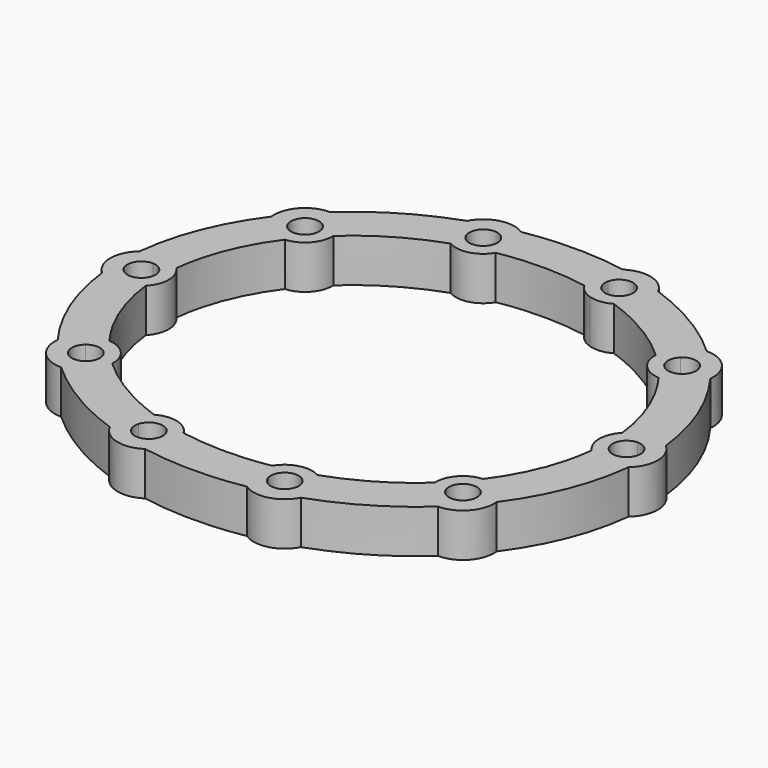
from build123d import *

# Parameters (mm, degrees)
F1_DEPTH = 3.5


with BuildPart() as f1:
    # F0 (on Top) → F1 (new body)
    with BuildSketch(Plane.XY):
        with BuildLine():
            add(Edge.make_bspline(
                [(17.9176777417, -1.5284816882), (18, -0.7659924616), (18, 0)],
                knots=[6.1875093004, 6.1875093004, 6.1875093004, 6.2831853072, 6.2831853072, 6.2831853072], degree=2, weights=[1, 0.9988559809, 1]))
            add(Edge.make_bspline(
                [(18, 0), (18, 0.7659924616), (17.9176777417, 1.5284816882)],
                knots=[0, 0, 0, 0.0956760068, 0.0956760068, 0.0956760068], degree=2, weights=[1, 0.9988559809, 1]))
            ThreePointArc((17.9176777417, 1.5284816882), (17.3, 0), (17.9176777417, -1.5284816882))
        make_face()
        with BuildLine():
            add(Edge.make_bspline(
                [(18, 0), (18, 0.7659924616), (17.9176777417, 1.5284816882)],
                knots=[0, 0, 0, 0.0956760068, 0.0956760068, 0.0956760068], degree=2, weights=[1, 0.9988559809, 1]))
            add(Edge.make_bspline(
                [(17.9176777417, -1.5284816882), (18, -0.7659924616), (18, 0)],
                knots=[6.1875093004, 6.1875093004, 6.1875093004, 6.2831853072, 6.2831853072, 6.2831853072], degree=2, weights=[1, 0.9988559809, 1]))
            add(Edge.make_bspline(
                [(15.0214595009, -8.8155084204), (17.4897174963, -5.4923559002), (17.9176777417, -1.5284816882)],
                knots=[5.6996600441, 5.6996600441, 5.6996600441, 6.1875093004, 6.1875093004, 6.1875093004], degree=2, weights=[1, 0.9703976022, 1]))
            add(Edge.make_bspline(
                [(12.9579027327, -11.1055188334), (14.108288617, -10.0449609858), (15.0214595009, -8.8155084204)],
                knots=[5.5160234188, 5.5160234188, 5.5160234188, 5.6996600441, 5.6996600441, 5.6996600441], degree=2, weights=[1, 0.9957876594, 1]))
            add(Edge.make_bspline(
                [(6.5641116037, -14.8981712717), (10.2272761366, -13.6229240841), (12.9579027327, -11.1055188334)],
                knots=[5.0856704323, 5.0856704323, 5.0856704323, 5.5160234188, 5.5160234188, 5.5160234188], degree=2, weights=[1, 0.9769387246, 1]))
            add(Edge.make_bspline(
                [(3.5634097577, -15.6833382916), (5.1022815412, -15.4070740686), (6.5641116037, -14.8981712717)],
                knots=[4.9116726299, 4.9116726299, 4.9116726299, 5.0856704323, 5.0856704323, 5.0856704323], degree=2, weights=[1, 0.9962179819, 1]))
            add(Edge.make_bspline(
                [(-3.5634097577, -15.6833382916), (0, -16.3230554133), (3.5634097577, -15.6833382916)],
                knots=[4.5131053308, 4.5131053308, 4.5131053308, 4.9116726299, 4.9116726299, 4.9116726299], degree=2, weights=[1, 0.9802086432, 1]))
            add(Edge.make_bspline(
                [(-6.5641116037, -14.8981712717), (-5.1022815412, -15.4070740686), (-3.5634097577, -15.6833382916)],
                knots=[4.3391075285, 4.3391075285, 4.3391075285, 4.5131053308, 4.5131053308, 4.5131053308], degree=2, weights=[1, 0.9962179819, 1]))
            add(Edge.make_bspline(
                [(-12.9579027327, -11.1055188334), (-10.2272761366, -13.6229240841), (-6.5641116037, -14.8981712717)],
                knots=[3.9087545419, 3.9087545419, 3.9087545419, 4.3391075285, 4.3391075285, 4.3391075285], degree=2, weights=[1, 0.9769387246, 1]))
            add(Edge.make_bspline(
                [(-15.0214595009, -8.8155084204), (-14.108288617, -10.0449609858), (-12.9579027327, -11.1055188334)],
                knots=[3.7251179166, 3.7251179166, 3.7251179166, 3.9087545419, 3.9087545419, 3.9087545419], degree=2, weights=[1, 0.9957876594, 1]))
            add(Edge.make_bspline(
                [(-17.9176777417, -1.5284816882), (-17.4897174963, -5.4923559002), (-15.0214595009, -8.8155084204)],
                knots=[3.2372686604, 3.2372686604, 3.2372686604, 3.7251179166, 3.7251179166, 3.7251179166], degree=2, weights=[1, 0.9703976022, 1]))
            add(Edge.make_bspline(
                [(-17.9176777417, 1.5284816882), (-18.0827004855, 0), (-17.9176777417, -1.5284816882)],
                knots=[3.0459166468, 3.0459166468, 3.0459166468, 3.2372686604, 3.2372686604, 3.2372686604], degree=2, weights=[1, 0.9954265412, 1]))
            add(Edge.make_bspline(
                [(-15.0214595009, 8.8155084204), (-17.4897174963, 5.4923559002), (-17.9176777417, 1.5284816882)],
                knots=[2.5580673905, 2.5580673905, 2.5580673905, 3.0459166468, 3.0459166468, 3.0459166468], degree=2, weights=[1, 0.9703976022, 1]))
            add(Edge.make_bspline(
                [(-12.9579027327, 11.1055188334), (-14.108288617, 10.0449609858), (-15.0214595009, 8.8155084204)],
                knots=[2.3744307652, 2.3744307652, 2.3744307652, 2.5580673905, 2.5580673905, 2.5580673905], degree=2, weights=[1, 0.9957876594, 1]))
            add(Edge.make_bspline(
                [(-6.5641116037, 14.8981712717), (-10.2272761366, 13.6229240841), (-12.9579027327, 11.1055188334)],
                knots=[1.9440777787, 1.9440777787, 1.9440777787, 2.3744307652, 2.3744307652, 2.3744307652], degree=2, weights=[1, 0.9769387246, 1]))
            add(Edge.make_bspline(
                [(-3.5634097577, 15.6833382916), (-5.1022815412, 15.4070740686), (-6.5641116037, 14.8981712717)],
                knots=[1.7700799764, 1.7700799764, 1.7700799764, 1.9440777787, 1.9440777787, 1.9440777787], degree=2, weights=[1, 0.9962179819, 1]))
            add(Edge.make_bspline(
                [(3.5634097577, 15.6833382916), (0, 16.3230554133), (-3.5634097577, 15.6833382916)],
                knots=[1.3715126772, 1.3715126772, 1.3715126772, 1.7700799764, 1.7700799764, 1.7700799764], degree=2, weights=[1, 0.9802086432, 1]))
            add(Edge.make_bspline(
                [(4.9945744172, 15.3717194589), (4.2861725259, 15.55358512), (3.5634097577, 15.6833382916)],
                knots=[1.2896300089, 1.2896300089, 1.2896300089, 1.3715126772, 1.3715126772, 1.3715126772], degree=2, weights=[1, 0.9991620206, 1]))
            Line((4.9945744172, 15.3717194589), (5.1111125116, 15.7303868336))
            ThreePointArc((5.1111125116, 15.7303868336), (4.4788764697, 16.247641173), (4.3632618671, 17.0562867863))
            add(Edge.make_bspline(
                [(4.3632618671, 17.0562867863), (0, 17.9552562546), (-4.3632618671, 17.0562867863)],
                knots=[1.3451287946, 1.3451287946, 1.3451287946, 1.796463859, 1.796463859, 1.796463859], degree=2, weights=[1, 0.9746449592, 1]))
            ThreePointArc((-4.3632618671, 17.0562867863), (-4.3411572816, 16.929153578), (-4.3337566303, 16.8003254145))
            ThreePointArc((-4.3337566303, 16.8003254145), (-5.3003624846, 15.6865317645), (-6.5391544874, 16.4866927147))
            add(Edge.make_bspline(
                [(-6.5391544874, 16.4866927147), (-11.1035556063, 15.028621514), (-14.3767828617, 11.8229512564)],
                knots=[1.9127637636, 1.9127637636, 1.9127637636, 2.3998182175, 2.3998182175, 2.3998182175], degree=2, weights=[1, 0.9704935031, 1]))
            ThreePointArc((-14.3767828617, 11.8229512564), (-14.1209684499, 11.4524934232), (-14.0308884413, 11.0113975023))
            ThreePointArc((-14.0308884413, 11.0113975023), (-14.6826870776, 9.9907577669), (-15.8828092758, 10.1527875208))
            add(Edge.make_bspline(
                [(-15.8828092758, 10.1527875208), (-19.1031132717, 6.0954067268), (-19.4597166867, 1.1242785485)],
                knots=[2.5226684132, 2.5226684132, 2.5226684132, 3.0773038895, 3.0773038895, 3.0773038895], degree=2, weights=[1, 0.9617932385, 1]))
            ThreePointArc((-19.4597166867, 1.1242785485), (-18.6903878313, 0.7811229969), (-18.375, 0))
            ThreePointArc((-18.375, 0), (-18.6903878313, -0.7811229969), (-19.4597166867, -1.1242785485))
            add(Edge.make_bspline(
                [(-19.4597166867, -1.1242785485), (-19.1031132717, -6.0954067268), (-15.8828092758, -10.1527875208)],
                knots=[3.2058814177, 3.2058814177, 3.2058814177, 3.7605168939, 3.7605168939, 3.7605168939], degree=2, weights=[1, 0.9617932385, 1]))
            ThreePointArc((-15.8828092758, -10.1527875208), (-14.6826870776, -9.9907577669), (-14.0308884413, -11.0113975023))
            ThreePointArc((-14.0308884413, -11.0113975023), (-14.1209684499, -11.4524934232), (-14.3767828617, -11.8229512564))
            add(Edge.make_bspline(
                [(-14.3767828617, -11.8229512564), (-11.1035556063, -15.028621514), (-6.5391544874, -16.4866927147)],
                knots=[3.8833670897, 3.8833670897, 3.8833670897, 4.3704215436, 4.3704215436, 4.3704215436], degree=2, weights=[1, 0.9704935031, 1]))
            ThreePointArc((-6.5391544874, -16.4866927147), (-5.3003624846, -15.6865317645), (-4.3337566303, -16.8003254145))
            ThreePointArc((-4.3337566303, -16.8003254145), (-4.3411572816, -16.929153578), (-4.3632618671, -17.0562867863))
            add(Edge.make_bspline(
                [(-4.3632618671, -17.0562867863), (0, -17.9552562546), (4.3632618671, -17.0562867863)],
                knots=[4.4867214482, 4.4867214482, 4.4867214482, 4.9380565126, 4.9380565126, 4.9380565126], degree=2, weights=[1, 0.9746449592, 1]))
            ThreePointArc((4.3632618671, -17.0562867863), (5.1738595774, -15.7119970315), (6.5391544874, -16.4866927147))
            add(Edge.make_bspline(
                [(6.5391544874, -16.4866927147), (11.1035556063, -15.028621514), (14.3767828617, -11.8229512564)],
                knots=[5.0543564172, 5.0543564172, 5.0543564172, 5.5414108711, 5.5414108711, 5.5414108711], degree=2, weights=[1, 0.9704935031, 1]))
            ThreePointArc((14.3767828617, -11.8229512564), (14.3203990411, -10.2580168136), (15.8828092758, -10.1527875208))
            add(Edge.make_bspline(
                [(15.8828092758, -10.1527875208), (19.1031132717, -6.0954067268), (19.4597166867, -1.1242785485)],
                knots=[5.6642610668, 5.6642610668, 5.6642610668, 6.2188965431, 6.2188965431, 6.2188965431], degree=2, weights=[1, 0.9617932385, 1]))
            ThreePointArc((19.4597166867, -1.1242785485), (18.375, 0), (19.4597166867, 1.1242785485))
            add(Edge.make_bspline(
                [(19.4597166867, 1.1242785485), (19.1031132717, 6.0954067268), (15.8828092758, 10.1527875208)],
                knots=[0.0642887641, 0.0642887641, 0.0642887641, 0.6189242404, 0.6189242404, 0.6189242404], degree=2, weights=[1, 0.9617932385, 1]))
            ThreePointArc((15.8828092758, 10.1527875208), (15.0212422242, 9.8944841681), (14.2457443226, 10.3501390935))
            Line((14.2457443226, 10.3501390935), (13.9368407211, 10.1257074899))
            add(Edge.make_bspline(
                [(15.0214595009, 8.8155084204), (14.5166626583, 9.4951443835), (13.9368407211, 10.1257074899)],
                knots=[0.583525263, 0.583525263, 0.583525263, 0.6852372416, 0.6852372416, 0.6852372416], degree=2, weights=[1, 0.9987071129, 1]))
            add(Edge.make_bspline(
                [(17.9176777417, 1.5284816882), (17.4897174963, 5.4923559002), (15.0214595009, 8.8155084204)],
                knots=[0.0956760068, 0.0956760068, 0.0956760068, 0.583525263, 0.583525263, 0.583525263], degree=2, weights=[1, 0.9703976022, 1]))
        make_face()
        with BuildLine():
            ThreePointArc((13.3760510537, 9.7182699473), (14.0976595024, 9.0826280726), (15.0214595009, 8.8155084204))
            add(Edge.make_bspline(
                [(15.0214595009, 8.8155084204), (14.5166626583, 9.4951443835), (13.9368407211, 10.1257074899)],
                knots=[0.583525263, 0.583525263, 0.583525263, 0.6852372416, 0.6852372416, 0.6852372416], degree=2, weights=[1, 0.9987071129, 1]))
            Line((13.9368407211, 10.1257074899), (13.3760510537, 9.7182699473))
        make_face()
        with BuildLine():
            add(Edge.make_bspline(
                [(12.9579027327, -11.1055188334), (14.108288617, -10.0449609858), (15.0214595009, -8.8155084204)],
                knots=[5.5160234188, 5.5160234188, 5.5160234188, 5.6996600441, 5.6996600441, 5.6996600441], degree=2, weights=[1, 0.9957876594, 1]))
            ThreePointArc((15.0214595009, -8.8155084204), (13.5215456234, -9.5386709311), (12.9579027327, -11.1055188334))
        make_face()
        with BuildLine():
            Line((13.3760510537, 9.7182699473), (13.9368407211, 10.1257074899))
            add(Edge.make_bspline(
                [(13.9368407211, 10.1257074899), (13.4699604962, 10.6334451693), (12.9579027327, 11.1055188334)],
                knots=[0.6852372416, 0.6852372416, 0.6852372416, 0.7671618883, 0.7671618883, 0.7671618883], degree=2, weights=[1, 0.9991611613, 1]))
            ThreePointArc((12.9579027327, 11.1055188334), (13.0494972112, 10.376483346), (13.3760510537, 9.7182699473))
        make_face()
        with BuildLine():
            add(Edge.make_bspline(
                [(13.9368407211, 10.1257074899), (13.4699604962, 10.6334451693), (12.9579027327, 11.1055188334)],
                knots=[0.6852372416, 0.6852372416, 0.6852372416, 0.7671618883, 0.7671618883, 0.7671618883], degree=2, weights=[1, 0.9991611613, 1]))
            Line((13.9368407211, 10.1257074899), (14.2457443226, 10.3501390935))
            ThreePointArc((14.2457443226, 10.3501390935), (14.0353149039, 11.1110967871), (14.3767828617, 11.8229512564))
            add(Edge.make_bspline(
                [(14.3767828617, 11.8229512564), (11.1035556063, 15.028621514), (6.5391544874, 16.4866927147)],
                knots=[0.7417744361, 0.7417744361, 0.7417744361, 1.22882889, 1.22882889, 1.22882889], degree=2, weights=[1, 0.9704935031, 1]))
            ThreePointArc((6.5391544874, 16.4866927147), (5.9852845562, 15.8061456806), (5.1111125116, 15.7303868336))
            Line((5.1111125116, 15.7303868336), (4.9945744172, 15.3717194589))
            add(Edge.make_bspline(
                [(6.5641116037, 14.8981712717), (5.7916200863, 15.1670965756), (4.9945744172, 15.3717194589)],
                knots=[1.1975148749, 1.1975148749, 1.1975148749, 1.2896300089, 1.2896300089, 1.2896300089], degree=2, weights=[1, 0.9989395377, 1]))
            add(Edge.make_bspline(
                [(12.9579027327, 11.1055188334), (10.2272761366, 13.6229240841), (6.5641116037, 14.8981712717)],
                knots=[0.7671618883, 0.7671618883, 0.7671618883, 1.1975148749, 1.1975148749, 1.1975148749], degree=2, weights=[1, 0.9769387246, 1]))
        make_face()
        with BuildLine():
            add(Edge.make_bspline(
                [(3.5634097577, -15.6833382916), (5.1022815412, -15.4070740686), (6.5641116037, -14.8981712717)],
                knots=[4.9116726299, 4.9116726299, 4.9116726299, 5.0856704323, 5.0856704323, 5.0856704323], degree=2, weights=[1, 0.9962179819, 1]))
            ThreePointArc((6.5641116037, -14.8981712718), (4.9018512412, -14.6719794869), (3.5634097577, -15.6833382916))
        make_face()
        with BuildLine():
            ThreePointArc((4.7789192427, 14.7080010786), (5.6917962826, 14.6127028418), (6.5641116037, 14.8981712718))
            add(Edge.make_bspline(
                [(6.5641116037, 14.8981712717), (5.7916200863, 15.1670965756), (4.9945744172, 15.3717194589)],
                knots=[1.1975148749, 1.1975148749, 1.1975148749, 1.2896300089, 1.2896300089, 1.2896300089], degree=2, weights=[1, 0.9989395377, 1]))
            Line((4.9945744172, 15.3717194589), (4.7789192427, 14.7080010786))
        make_face()
        with BuildLine():
            add(Edge.make_bspline(
                [(14.3767828617, 11.8229512564), (11.1035556063, 15.028621514), (6.5391544874, 16.4866927147)],
                knots=[0.7417744361, 0.7417744361, 0.7417744361, 1.22882889, 1.22882889, 1.22882889], degree=2, weights=[1, 0.9704935031, 1]))
            ThreePointArc((14.3767828617, 11.8229512564), (15.2555877261, 12.1319710397), (16.06603256, 11.6726559111))
            Line((16.06603256, 11.6726559111), (16.5770547092, 12.0439352353))
            add(Edge.make_bspline(
                [(16.5770547092, 12.0439352353), (15.897962477, 12.8109634173), (15.1361324024, 13.5113194409)],
                knots=[0.6759759799, 0.6759759799, 0.6759759799, 0.7780428717, 0.7780428717, 0.7780428717], degree=2, weights=[1, 0.9986980763, 1]))
            add(Edge.make_bspline(
                [(15.1361324024, 13.5113194409), (11.9335945642, 16.455436168), (7.6791841945, 17.9491080015)],
                knots=[0.7780428717, 0.7780428717, 0.7780428717, 1.2010559415, 1.2010559415, 1.2010559415], degree=2, weights=[1, 0.9777157528, 1]))
            add(Edge.make_bspline(
                [(7.6791841945, 17.9491080015), (6.8516175805, 18.2396565932), (6.0001876976, 18.4666788968)],
                knots=[1.2010559415, 1.2010559415, 1.2010559415, 1.2845411506, 1.2845411506, 1.2845411506], degree=2, weights=[1, 0.999128904, 1]))
            Line((6.0001876976, 18.4666788968), (5.806400749, 17.8702639953))
            ThreePointArc((5.806400749, 17.8702639953), (6.368900749, 17.4615838233), (6.5837566303, 16.8003254145))
            ThreePointArc((6.5837566303, 16.8003254145), (6.5725502802, 16.6419312688), (6.5391544874, 16.4866927147))
        make_face()
        with BuildLine():
            ThreePointArc((16.2808884413, 11.0113975023), (16.1765281767, 10.5381961386), (15.8828092758, 10.1527875208))
            add(Edge.make_bspline(
                [(19.4597166867, 1.1242785485), (19.1031132717, 6.0954067268), (15.8828092758, 10.1527875208)],
                knots=[0.0642887641, 0.0642887641, 0.0642887641, 0.6189242404, 0.6189242404, 0.6189242404], degree=2, weights=[1, 0.9617932385, 1]))
            ThreePointArc((19.4597166867, 1.1242785485), (20.2811229969, 0.8096121687), (20.625, 0))
            ThreePointArc((20.625, 0), (20.2811229969, -0.8096121687), (19.4597166867, -1.1242785485))
            add(Edge.make_bspline(
                [(15.8828092758, -10.1527875208), (19.1031132717, -6.0954067268), (19.4597166867, -1.1242785485)],
                knots=[5.6642610668, 5.6642610668, 5.6642610668, 6.2188965431, 6.2188965431, 6.2188965431], degree=2, weights=[1, 0.9617932385, 1]))
            ThreePointArc((15.8828092758, -10.1527875208), (16.1765281767, -10.5381961386), (16.2808884413, -11.0113975023))
            ThreePointArc((16.2808884413, -11.0113975023), (15.5969843622, -12.0463174937), (14.3767828617, -11.8229512564))
            add(Edge.make_bspline(
                [(6.5391544874, -16.4866927147), (11.1035556063, -15.028621514), (14.3767828617, -11.8229512564)],
                knots=[5.0543564172, 5.0543564172, 5.0543564172, 5.5414108711, 5.5414108711, 5.5414108711], degree=2, weights=[1, 0.9704935031, 1]))
            ThreePointArc((6.5391544874, -16.4866927147), (6.5725502802, -16.6419312688), (6.5837566303, -16.8003254145))
            ThreePointArc((6.5837566303, -16.8003254145), (5.5875847938, -17.9179247632), (4.3632618671, -17.0562867863))
            add(Edge.make_bspline(
                [(-4.3632618671, -17.0562867863), (0, -17.9552562546), (4.3632618671, -17.0562867863)],
                knots=[4.4867214482, 4.4867214482, 4.4867214482, 4.9380565126, 4.9380565126, 4.9380565126], degree=2, weights=[1, 0.9746449592, 1]))
            ThreePointArc((-4.3632618671, -17.0562867863), (-5.7436536832, -17.8886537975), (-6.5391544874, -16.4866927147))
            add(Edge.make_bspline(
                [(-14.3767828617, -11.8229512564), (-11.1035556063, -15.028621514), (-6.5391544874, -16.4866927147)],
                knots=[3.8833670897, 3.8833670897, 3.8833670897, 4.3704215436, 4.3704215436, 4.3704215436], degree=2, weights=[1, 0.9704935031, 1]))
            ThreePointArc((-14.3767828617, -11.8229512564), (-15.9913778415, -11.764778191), (-15.8828092758, -10.1527875208))
            add(Edge.make_bspline(
                [(-19.4597166867, -1.1242785485), (-19.1031132717, -6.0954067268), (-15.8828092758, -10.1527875208)],
                knots=[3.2058814177, 3.2058814177, 3.2058814177, 3.7605168939, 3.7605168939, 3.7605168939], degree=2, weights=[1, 0.9617932385, 1]))
            ThreePointArc((-19.4597166867, -1.1242785485), (-20.625, 0), (-19.4597166867, 1.1242785485))
            add(Edge.make_bspline(
                [(-15.8828092758, 10.1527875208), (-19.1031132717, 6.0954067268), (-19.4597166867, 1.1242785485)],
                knots=[2.5226684132, 2.5226684132, 2.5226684132, 3.0773038895, 3.0773038895, 3.0773038895], degree=2, weights=[1, 0.9617932385, 1]))
            ThreePointArc((-15.8828092758, 10.1527875208), (-15.9913778415, 11.764778191), (-14.3767828617, 11.8229512564))
            add(Edge.make_bspline(
                [(-6.5391544874, 16.4866927147), (-11.1035556063, 15.028621514), (-14.3767828617, 11.8229512564)],
                knots=[1.9127637636, 1.9127637636, 1.9127637636, 2.3998182175, 2.3998182175, 2.3998182175], degree=2, weights=[1, 0.9704935031, 1]))
            ThreePointArc((-6.5391544874, 16.4866927147), (-5.7436536832, 17.8886537975), (-4.3632618671, 17.0562867863))
            add(Edge.make_bspline(
                [(4.3632618671, 17.0562867863), (0, 17.9552562546), (-4.3632618671, 17.0562867863)],
                knots=[1.3451287946, 1.3451287946, 1.3451287946, 1.796463859, 1.796463859, 1.796463859], degree=2, weights=[1, 0.9746449592, 1]))
            ThreePointArc((4.3632618671, 17.0562867863), (4.9060723888, 17.7802055751), (5.806400749, 17.8702639953))
            Line((5.806400749, 17.8702639953), (6.0001876976, 18.4666788968))
            add(Edge.make_bspline(
                [(6.0001876976, 18.4666788968), (5.054591039, 18.7188095021), (4.0872893489, 18.8905592521)],
                knots=[1.2845411506, 1.2845411506, 1.2845411506, 1.3772471262, 1.3772471262, 1.3772471262], degree=2, weights=[1, 0.9989258926, 1]))
            add(Edge.make_bspline(
                [(4.0872893489, 18.8905592521), (0, 19.6162800187), (-4.0872893489, 18.8905592521)],
                knots=[1.3772471262, 1.3772471262, 1.3772471262, 1.7643455274, 1.7643455274, 1.7643455274], degree=2, weights=[1, 0.9813277534, 1]))
            add(Edge.make_bspline(
                [(-4.0872893489, 18.8905592521), (-5.9291328688, 18.5635297768), (-7.6791841945, 17.9491080015)],
                knots=[1.7643455274, 1.7643455274, 1.7643455274, 1.9405367121, 1.9405367121, 1.9405367121], degree=2, weights=[1, 0.9961220923, 1]))
            add(Edge.make_bspline(
                [(-7.6791841945, 17.9491080015), (-11.9335945642, 16.455436168), (-15.1361324024, 13.5113194409)],
                knots=[1.9405367121, 1.9405367121, 1.9405367121, 2.3635497819, 2.3635497819, 2.3635497819], degree=2, weights=[1, 0.9777157528, 1]))
            add(Edge.make_bspline(
                [(-15.1361324024, 13.5113194409), (-16.5317231543, 12.2283425381), (-17.6403504529, 10.7331017735)],
                knots=[2.3635497819, 2.3635497819, 2.3635497819, 2.5501445486, 2.5501445486, 2.5501445486], degree=2, weights=[1, 0.9956509552, 1]))
            add(Edge.make_bspline(
                [(-17.6403504529, 10.7331017735), (-20.6256967553, 6.7066706246), (-21.1484700681, 1.8795069658)],
                knots=[2.5501445486, 2.5501445486, 2.5501445486, 3.0438001315, 3.0438001315, 3.0438001315], degree=2, weights=[1, 0.9696923623, 1]))
            add(Edge.make_bspline(
                [(-21.1484700681, 1.8795069658), (-21.3520173585, 0), (-21.1484700681, -1.8795069658)],
                knots=[3.0438001315, 3.0438001315, 3.0438001315, 3.2393851757, 3.2393851757, 3.2393851757], degree=2, weights=[1, 0.9952221209, 1]))
            add(Edge.make_bspline(
                [(-21.1484700681, -1.8795069658), (-20.6256967553, -6.7066706246), (-17.6403504529, -10.7331017735)],
                knots=[3.2393851757, 3.2393851757, 3.2393851757, 3.7330407586, 3.7330407586, 3.7330407586], degree=2, weights=[1, 0.9696923623, 1]))
            add(Edge.make_bspline(
                [(-17.6403504529, -10.7331017735), (-16.5317231543, -12.2283425381), (-15.1361324024, -13.5113194409)],
                knots=[3.7330407586, 3.7330407586, 3.7330407586, 3.9196355253, 3.9196355253, 3.9196355253], degree=2, weights=[1, 0.9956509552, 1]))
            add(Edge.make_bspline(
                [(-15.1361324024, -13.5113194409), (-11.9335945642, -16.455436168), (-7.6791841945, -17.9491080015)],
                knots=[3.9196355253, 3.9196355253, 3.9196355253, 4.3426485951, 4.3426485951, 4.3426485951], degree=2, weights=[1, 0.9777157528, 1]))
            add(Edge.make_bspline(
                [(-7.6791841945, -17.9491080015), (-5.9291328688, -18.5635297768), (-4.0872893489, -18.8905592521)],
                knots=[4.3426485951, 4.3426485951, 4.3426485951, 4.5188397798, 4.5188397798, 4.5188397798], degree=2, weights=[1, 0.9961220923, 1]))
            add(Edge.make_bspline(
                [(-4.0872893489, -18.8905592521), (0, -19.6162800187), (4.0872893489, -18.8905592521)],
                knots=[4.5188397798, 4.5188397798, 4.5188397798, 4.905938181, 4.905938181, 4.905938181], degree=2, weights=[1, 0.9813277534, 1]))
            add(Edge.make_bspline(
                [(4.0872893489, -18.8905592521), (5.9291328688, -18.5635297768), (7.6791841945, -17.9491080015)],
                knots=[4.905938181, 4.905938181, 4.905938181, 5.0821293656, 5.0821293656, 5.0821293656], degree=2, weights=[1, 0.9961220923, 1]))
            add(Edge.make_bspline(
                [(7.6791841945, -17.9491080015), (11.9335945642, -16.455436168), (15.1361324024, -13.5113194409)],
                knots=[5.0821293656, 5.0821293656, 5.0821293656, 5.5051424355, 5.5051424355, 5.5051424355], degree=2, weights=[1, 0.9777157528, 1]))
            add(Edge.make_bspline(
                [(15.1361324024, -13.5113194409), (16.5317231543, -12.2283425381), (17.6403504529, -10.7331017735)],
                knots=[5.5051424355, 5.5051424355, 5.5051424355, 5.6917372022, 5.6917372022, 5.6917372022], degree=2, weights=[1, 0.9956509552, 1]))
            add(Edge.make_bspline(
                [(17.6403504529, -10.7331017735), (20.6256967553, -6.7066706246), (21.1484700681, -1.8795069658)],
                knots=[5.6917372022, 5.6917372022, 5.6917372022, 6.1853927851, 6.1853927851, 6.1853927851], degree=2, weights=[1, 0.9696923623, 1]))
            add(Edge.make_bspline(
                [(21.1484700681, -1.8795069658), (21.25, -0.9420038732), (21.25, 0)],
                knots=[6.1853927851, 6.1853927851, 6.1853927851, 6.2831853072, 6.2831853072, 6.2831853072], degree=2, weights=[1, 0.998804816, 1]))
            add(Edge.make_bspline(
                [(21.25, 0), (21.25, 0.9420038732), (21.1484700681, 1.8795069658)],
                knots=[0, 0, 0, 0.0977925221, 0.0977925221, 0.0977925221], degree=2, weights=[1, 0.998804816, 1]))
            add(Edge.make_bspline(
                [(21.1484700681, 1.8795069658), (20.6256967553, 6.7066706246), (17.6403504529, 10.7331017735)],
                knots=[0.0977925221, 0.0977925221, 0.0977925221, 0.591448105, 0.591448105, 0.591448105], degree=2, weights=[1, 0.9696923623, 1]))
            add(Edge.make_bspline(
                [(17.6403504529, 10.7331017735), (17.1392992658, 11.4088853854), (16.5770547092, 12.0439352353)],
                knots=[0.591448105, 0.591448105, 0.591448105, 0.6759759799, 0.6759759799, 0.6759759799], degree=2, weights=[1, 0.9991070127, 1]))
            Line((16.5770547092, 12.0439352353), (16.06603256, 11.6726559111))
            ThreePointArc((16.06603256, 11.6726559111), (16.2258270221, 11.359041621), (16.2808884413, 11.0113975023))
        make_face()
        with BuildLine():
            ThreePointArc((3.5634097577, 15.6833382916), (4.0819072691, 15.0844332743), (4.7789192427, 14.7080010786))
            Line((4.7789192427, 14.7080010786), (4.9945744172, 15.3717194589))
            add(Edge.make_bspline(
                [(4.9945744172, 15.3717194589), (4.2861725259, 15.55358512), (3.5634097577, 15.6833382916)],
                knots=[1.2896300089, 1.2896300089, 1.2896300089, 1.3715126772, 1.3715126772, 1.3715126772], degree=2, weights=[1, 0.9991620206, 1]))
        make_face()
        with BuildLine():
            add(Edge.make_bspline(
                [(-6.5641116037, -14.8981712717), (-5.1022815412, -15.4070740686), (-3.5634097577, -15.6833382916)],
                knots=[4.3391075285, 4.3391075285, 4.3391075285, 4.5131053308, 4.5131053308, 4.5131053308], degree=2, weights=[1, 0.9962179819, 1]))
            ThreePointArc((-3.5634097577, -15.6833382916), (-4.9018512412, -14.6719794869), (-6.5641116037, -14.8981712718))
        make_face()
        with BuildLine():
            Line((17.1784309272, 12.480860633), (16.5770547092, 12.0439352353))
            add(Edge.make_bspline(
                [(17.6403504529, 10.7331017735), (17.1392992658, 11.4088853854), (16.5770547092, 12.0439352353)],
                knots=[0.591448105, 0.591448105, 0.591448105, 0.6759759799, 0.6759759799, 0.6759759799], degree=2, weights=[1, 0.9991070127, 1]))
            ThreePointArc((17.6403504529, 10.7331017735), (17.572898504, 11.6501950891), (17.1784309272, 12.480860633))
        make_face()
        with BuildLine():
            add(Edge.make_bspline(
                [(16.5770547092, 12.0439352353), (15.897962477, 12.8109634173), (15.1361324024, 13.5113194409)],
                knots=[0.6759759799, 0.6759759799, 0.6759759799, 0.7780428717, 0.7780428717, 0.7780428717], degree=2, weights=[1, 0.9986980763, 1]))
            Line((16.5770547092, 12.0439352353), (17.1784309272, 12.480860633))
            ThreePointArc((17.1784309272, 12.480860633), (16.2820543824, 13.2433809864), (15.1361324024, 13.5113194409))
        make_face()
        with BuildLine():
            ThreePointArc((-6.5641116037, 14.8981712718), (-4.9018512412, 14.6719794869), (-3.5634097577, 15.6833382916))
            add(Edge.make_bspline(
                [(-3.5634097577, 15.6833382916), (-5.1022815412, 15.4070740686), (-6.5641116037, 14.8981712717)],
                knots=[1.7700799764, 1.7700799764, 1.7700799764, 1.9440777787, 1.9440777787, 1.9440777787], degree=2, weights=[1, 0.9962179819, 1]))
        make_face()
        with BuildLine():
            add(Edge.make_bspline(
                [(-15.0214595009, -8.8155084204), (-14.108288617, -10.0449609858), (-12.9579027327, -11.1055188334)],
                knots=[3.7251179166, 3.7251179166, 3.7251179166, 3.9087545419, 3.9087545419, 3.9087545419], degree=2, weights=[1, 0.9957876594, 1]))
            ThreePointArc((-12.9579027327, -11.1055188334), (-13.5215456234, -9.5386709311), (-15.0214595009, -8.8155084204))
        make_face()
        with BuildLine():
            ThreePointArc((21.1484700681, -1.8795069658), (22, 0), (21.1484700681, 1.8795069658))
            add(Edge.make_bspline(
                [(21.25, 0), (21.25, 0.9420038732), (21.1484700681, 1.8795069658)],
                knots=[0, 0, 0, 0.0977925221, 0.0977925221, 0.0977925221], degree=2, weights=[1, 0.998804816, 1]))
            add(Edge.make_bspline(
                [(21.1484700681, -1.8795069658), (21.25, -0.9420038732), (21.25, 0)],
                knots=[6.1853927851, 6.1853927851, 6.1853927851, 6.2831853072, 6.2831853072, 6.2831853072], degree=2, weights=[1, 0.998804816, 1]))
        make_face()
        with BuildLine():
            add(Edge.make_bspline(
                [(7.6791841945, 17.9491080015), (6.8516175805, 18.2396565932), (6.0001876976, 18.4666788968)],
                knots=[1.2010559415, 1.2010559415, 1.2010559415, 1.2845411506, 1.2845411506, 1.2845411506], degree=2, weights=[1, 0.999128904, 1]))
            ThreePointArc((7.6791841945, 17.9491080015), (7.076468242, 18.706370834), (6.2312991162, 19.1779667052))
            Line((6.2312991162, 19.1779667052), (6.0001876976, 18.4666788968))
        make_face()
        with BuildLine():
            add(Edge.make_bspline(
                [(6.0001876976, 18.4666788968), (5.054591039, 18.7188095021), (4.0872893489, 18.8905592521)],
                knots=[1.2845411506, 1.2845411506, 1.2845411506, 1.3772471262, 1.3772471262, 1.3772471262], degree=2, weights=[1, 0.9989258926, 1]))
            Line((6.0001876976, 18.4666788968), (6.2312991162, 19.1779667052))
            ThreePointArc((6.2312991162, 19.1779667052), (5.1265993051, 19.2781614686), (4.0872893489, 18.8905592521))
        make_face()
        with BuildLine():
            ThreePointArc((-15.0214595009, 8.8155084204), (-13.5215456234, 9.5386709311), (-12.9579027327, 11.1055188334))
            add(Edge.make_bspline(
                [(-12.9579027327, 11.1055188334), (-14.108288617, 10.0449609858), (-15.0214595009, 8.8155084204)],
                knots=[2.3744307652, 2.3744307652, 2.3744307652, 2.5580673905, 2.5580673905, 2.5580673905], degree=2, weights=[1, 0.9957876594, 1]))
        make_face()
        with BuildLine():
            add(Edge.make_bspline(
                [(-17.9176777417, 1.5284816882), (-18.0827004855, 0), (-17.9176777417, -1.5284816882)],
                knots=[3.0459166468, 3.0459166468, 3.0459166468, 3.2372686604, 3.2372686604, 3.2372686604], degree=2, weights=[1, 0.9954265412, 1]))
            ThreePointArc((-17.9176777417, -1.5284816882), (-17.3, 0), (-17.9176777417, 1.5284816882))
        make_face()
        with BuildLine():
            ThreePointArc((15.1361324024, -13.5113194409), (17.012852963, -12.6852203021), (17.6403504529, -10.7331017735))
            add(Edge.make_bspline(
                [(15.1361324024, -13.5113194409), (16.5317231543, -12.2283425381), (17.6403504529, -10.7331017735)],
                knots=[5.5051424355, 5.5051424355, 5.5051424355, 5.6917372022, 5.6917372022, 5.6917372022], degree=2, weights=[1, 0.9956509552, 1]))
        make_face()
        with BuildLine():
            add(Edge.make_bspline(
                [(-4.0872893489, 18.8905592521), (-5.9291328688, 18.5635297768), (-7.6791841945, 17.9491080015)],
                knots=[1.7643455274, 1.7643455274, 1.7643455274, 1.9405367121, 1.9405367121, 1.9405367121], degree=2, weights=[1, 0.9961220923, 1]))
            ThreePointArc((-4.0872893489, 18.8905592521), (-6.0926067741, 19.2186376349), (-7.6791841945, 17.9491080015))
        make_face()
        with BuildLine():
            ThreePointArc((4.0872893489, -18.8905592521), (6.0926067741, -19.2186376349), (7.6791841945, -17.9491080015))
            add(Edge.make_bspline(
                [(4.0872893489, -18.8905592521), (5.9291328688, -18.5635297768), (7.6791841945, -17.9491080015)],
                knots=[4.905938181, 4.905938181, 4.905938181, 5.0821293656, 5.0821293656, 5.0821293656], degree=2, weights=[1, 0.9961220923, 1]))
        make_face()
        with BuildLine():
            add(Edge.make_bspline(
                [(-15.1361324024, 13.5113194409), (-16.5317231543, 12.2283425381), (-17.6403504529, 10.7331017735)],
                knots=[2.3635497819, 2.3635497819, 2.3635497819, 2.5501445486, 2.5501445486, 2.5501445486], degree=2, weights=[1, 0.9956509552, 1]))
            ThreePointArc((-15.1361324024, 13.5113194409), (-17.012852963, 12.6852203021), (-17.6403504529, 10.7331017735))
        make_face()
        with BuildLine():
            ThreePointArc((-7.6791841945, -17.9491080015), (-6.0926067741, -19.2186376349), (-4.0872893489, -18.8905592521))
            add(Edge.make_bspline(
                [(-7.6791841945, -17.9491080015), (-5.9291328688, -18.5635297768), (-4.0872893489, -18.8905592521)],
                knots=[4.3426485951, 4.3426485951, 4.3426485951, 4.5188397798, 4.5188397798, 4.5188397798], degree=2, weights=[1, 0.9961220923, 1]))
        make_face()
        with BuildLine():
            add(Edge.make_bspline(
                [(-21.1484700681, 1.8795069658), (-21.3520173585, 0), (-21.1484700681, -1.8795069658)],
                knots=[3.0438001315, 3.0438001315, 3.0438001315, 3.2393851757, 3.2393851757, 3.2393851757], degree=2, weights=[1, 0.9952221209, 1]))
            ThreePointArc((-21.1484700681, 1.8795069658), (-22, 0), (-21.1484700681, -1.8795069658))
        make_face()
        with BuildLine():
            ThreePointArc((-17.6403504529, -10.7331017735), (-17.012852963, -12.6852203021), (-15.1361324024, -13.5113194409))
            add(Edge.make_bspline(
                [(-17.6403504529, -10.7331017735), (-16.5317231543, -12.2283425381), (-15.1361324024, -13.5113194409)],
                knots=[3.7330407586, 3.7330407586, 3.7330407586, 3.9196355253, 3.9196355253, 3.9196355253], degree=2, weights=[1, 0.9956509552, 1]))
        make_face()
    extrude(amount=F1_DEPTH)


solid = f1.part
